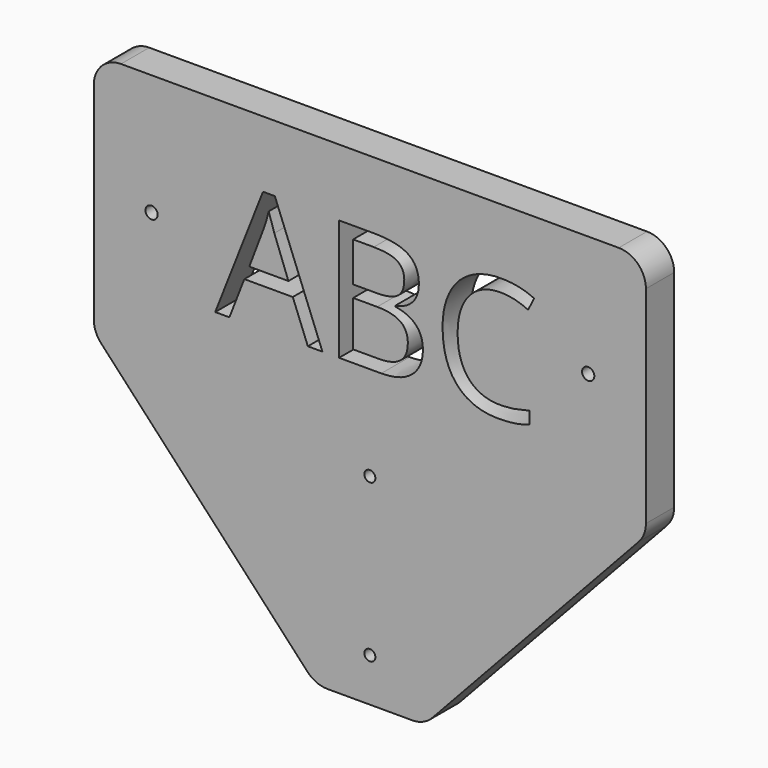
from build123d import *

# Parameters (mm, degrees)
F1_DEPTH     = 13
F2_R         = 2.02162981
F2_R_2       = 2.25
F3_DEPTH     = 25
F4_R         = 10
F5_TEXT_SIZE = 62.3660369052
F6_DEPTH     = 25


# Not quite as in the source:
# - Text() gives the source's letters only with a copy of the font that has no kerning and outlines rounded to 1/6400 em; it was checked with that copy


with BuildPart() as f1:
    # F0 (on Front) → F1 (new body)
    with BuildSketch(Plane.XZ):
        Polygon((-20, 0), (0, 0), (20, 0), (101.6, 87.8), (101.6, 177.8), (0, 177.8), (-101.6, 177.8), (-101.6, 87.8), align=None)
    extrude(amount=F1_DEPTH)

    # F2 (on face) → F3 (cut)
    with BuildSketch(Plane.XZ.offset(13)):
        with Locations((0, 74)):
            Circle(F2_R)
        with Locations((0, 16.02162981)):
            Circle(F2_R)
        with Locations((-80.35, 133.3)):
            Circle(F2_R_2)
        with Locations((80.35, 133.3)):
            Circle(F2_R_2)
    extrude(amount=-F3_DEPTH, mode=Mode.SUBTRACT)

    # F4
    f4_edges = [f1.edges().sort_by_distance(p)[0] for p in [
        (101.6, -6.5, 177.8),
        (101.6, -6.5, 87.8),
        (-20, -6.5, 0),
        (20, -6.5, 0),
        (-101.6, -6.5, 87.8),
        (-101.6, -6.5, 177.8),
    ]]
    fillet(f4_edges, radius=F4_R)

    # F5 (on face) → F6 (cut)
    with BuildSketch(Plane.XZ.offset(13)):
        with Locations((-56.9307664409, 108.6888611317)):
            Text('ABC', F5_TEXT_SIZE, font='Open Sans', text_align=(TextAlign.LEFT, TextAlign.BOTTOM))
    extrude(amount=-F6_DEPTH, mode=Mode.SUBTRACT)


solid = f1.part
